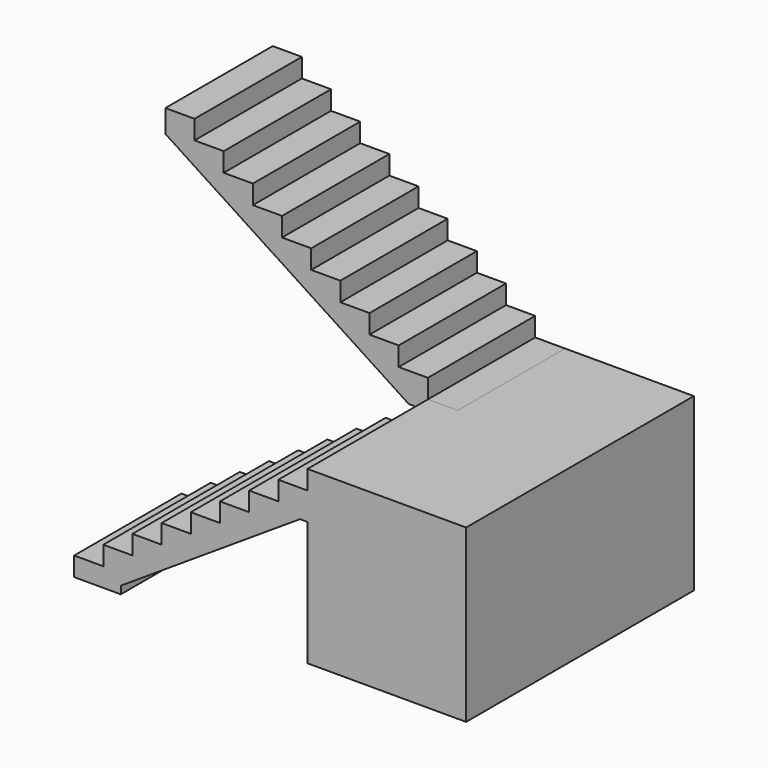
from build123d import *

# Parameters (mm, degrees)
F1_DEPTH = 1150
F4_DEPTH = 1150
F5_W     = 1360
F5_H     = 2440
F6_DEPTH = 1467


with BuildPart() as f1:
    # F0 (on Front) → F1 (new body)
    with BuildSketch(Plane.XZ):
        Polygon((0, 163), (0, 0), (400, 0), (400, 65.6668404071), (1935.7870545904, 1067), (2250, 1067), (2250, 1467), (2000, 1467), (2000, 1304), (1750, 1304), (1750, 1141), (1500, 1141), (1500, 978), (1250, 978), (1250, 815), (1000, 815), (1000, 652), (750, 652), (750, 489), (500, 489), (500, 326), (250, 326), (250, 163), align=None)
    extrude(amount=F1_DEPTH)

    # F5 (on Top) → F6 (join)
    with BuildSketch(Plane.XY):
        with Locations((2680, 70)):
            Rectangle(F5_W, F5_H)
    extrude(amount=F6_DEPTH)


with BuildPart() as f4:
    # F3 (on offset) → F4 (new body)
    with BuildSketch(Plane.XZ.offset(-140)):
        Polygon((2000, 1630), (1750, 1630), (1750, 1793), (1500, 1793), (1500, 1956), (1250, 1956), (1250, 2119), (1000, 2119), (1000, 2282), (750, 2282), (750, 2445), (500, 2445), (500, 2608), (250, 2608), (250, 2771), (0, 2771), (0, 2934), (-250, 2934), (-250, 2738.8668404071), (1836.1503300429, 1378.6968252191), (2256.0992240906, 1378.6968252191), (2256.0992240906, 1467), (2000, 1467), align=None)
    extrude(amount=-F4_DEPTH)


solid = Compound([f1.part, f4.part])
